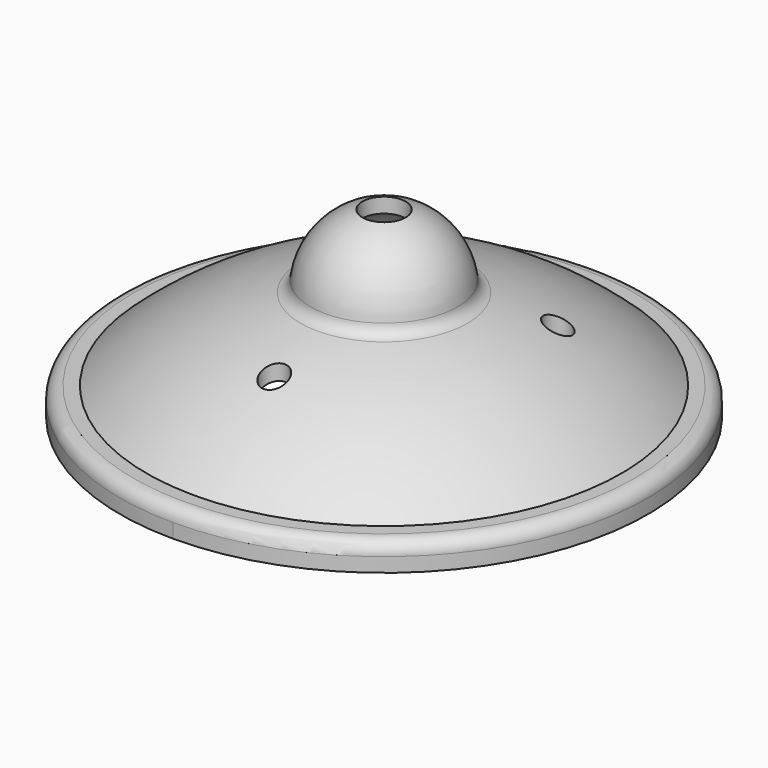
from build123d import *

# Parameters (mm, degrees)
F2_R      = 20
F3_DEPTH  = 25
F4_R      = 2.5
F5_DEPTH  = 25
F7_W      = 12
F7_H      = 6.6
F8_DEPTH  = 60
F9_R      = 4.1
F9_R_2    = 2.5
F10_DEPTH = 15


# Not quite as in the source:
# - a fillet or chamfer that OpenCascade refuses, or shapes differently, is made with other operations: its cross-section is extruded or revolved along the edge and cut away or added
# - a feature names something its author has since deleted; it is built from what else it names


with BuildPart() as f1:
    # F0 (on Right) → F1 (revolve)
    with BuildSketch(Plane.YZ):
        with BuildLine():
            Line((-47, 0.8), (-47, 2))
            Line((-47, 2), (-47, 4))
            Line((-47, 4), (-42, 4))
            Line((-42, 4), (-42, 6))
            ThreePointArc((-42, 6), (-27.3273562245, 14.6498550341), (-11, 19.5))
            Line((-11, 19.5), (-2.5, 19.5))
            Line((-2.5, 19.5), (-2.5, 22.5))
            Line((-2.5, 22.5), (-11, 22.5))
            ThreePointArc((-11, 22.5), (-7.9199859369, 30.2852233625), (0, 33))
            Line((0, 33), (0, 36))
            ThreePointArc((0, 36), (-9.9253616904, 31.873751261), (-14, 21.9270907164))
            ThreePointArc((-14, 21.9270907164), (-30.5537547763, 16.0145412775), (-45, 6))
            Line((-45, 6), (-50, 6))
            Line((-50, 6), (-50, 0.8))
            Line((-50, 0.8), (-47, 0.8))
        make_face()
    revolve(axis=Axis((0, 0, -9), (0, 0, -1)))

    # F2 (on Top) → F3 (cut)
    with BuildSketch(Plane.XY):
        Circle(F2_R)
    extrude(amount=-F3_DEPTH, mode=Mode.SUBTRACT)

    # F4 (on Top) → F5 (cut)
    with BuildSketch(Plane.XY):
        with Locations((0, -26)):
            Circle(F4_R)
        with Locations((-22.5166604984, 13)):
            Circle(F4_R)
        with Locations((22.5166604984, 13)):
            Circle(F4_R)
    extrude(amount=F5_DEPTH, mode=Mode.SUBTRACT)

    # F6: fillet of radius 5 on 1 edges, made by hand

    # F6_s1 → F6_t2 (revolve)
    with BuildSketch(Plane.YZ):
        with BuildLine():
            ThreePointArc((-42, 4), (-41.3412296148, 5.9882107587), (-39.9258684636, 7.532138624))
            ThreePointArc((-39.9258684636, 7.532138624), (-40.9699899366, 6.7756209672), (-42, 6))
            Line((-42, 6), (-42, 4))
        make_face()
    revolve(axis=Axis((0, 0, 6), (0, 0, -1)))

    # F7 (on Front) → F8 (cut)
    with BuildSketch(Plane.XZ):
        with Locations((0, 0.3)):
            Rectangle(F7_W, F7_H)
    extrude(amount=-F8_DEPTH, mode=Mode.SUBTRACT)

    # F9 (on face) → F10 (cut)
    with BuildSketch(Plane.XY.offset(22.5)):
        Circle(F9_R)
        Circle(F9_R_2, mode=Mode.SUBTRACT)
        Circle(F9_R_2)
    extrude(amount=F10_DEPTH, mode=Mode.SUBTRACT)

    # F11: fillet of radius 2.5 on 2 edges, made by hand

    # F11_s1 → F11_t2 (revolve)
    with BuildSketch(Plane.YZ):
        with BuildLine():
            ThreePointArc((-15.7934154108, 21.5162006837), (-14.513888258, 22.2873217713), (-13.902565029, 23.6504436939))
            ThreePointArc((-13.902565029, 23.6504436939), (-13.9778675149, 22.7902702686), (-14, 21.9270907164))
            ThreePointArc((-14, 21.9270907164), (-14.8981182002, 21.7278020994), (-15.7934154108, 21.5162006837))
        make_face()
    revolve(axis=Axis((0, 0, 21.9270907164), (0, 0, -1)))

    # F11_s3 → F11_t4 (revolve, cut)
    with BuildSketch(Plane.YZ):
        with BuildLine():
            ThreePointArc((-47.5, 6), (-49.267766953, 5.267766953), (-50, 3.5))
            Line((-50, 3.5), (-50, 6))
            Line((-50, 6), (-47.5, 6))
        make_face()
    revolve(axis=Axis((0, 0, 6), (0, 0, -1)), mode=Mode.SUBTRACT)


solid = f1.part
